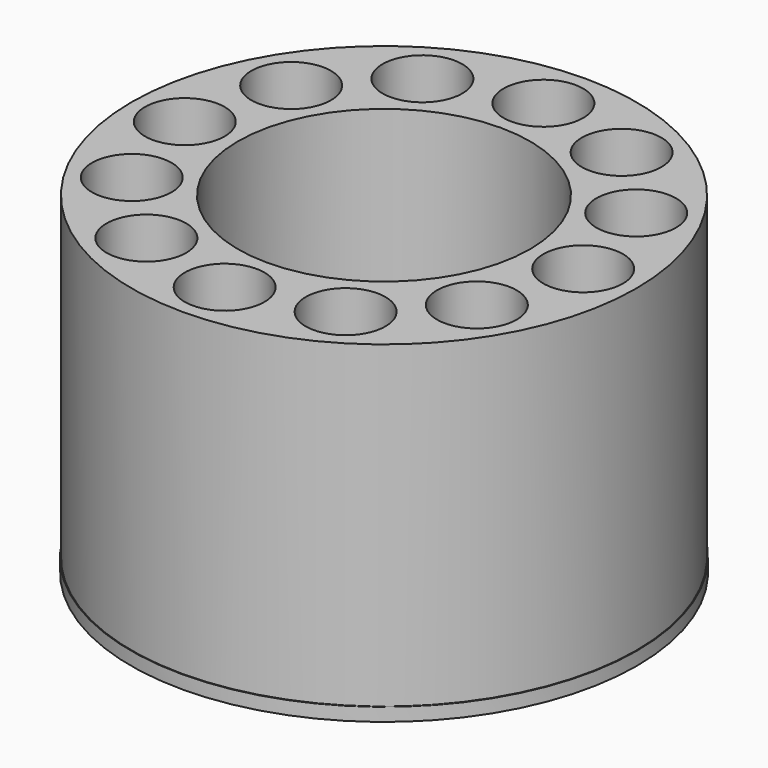
from build123d import *

# Parameters (mm, degrees)
F0_R     = 30.1625
F0_R_2   = 4.7625
F0_R_3   = 17.4625
F1_DEPTH = 38.1
F2_R     = 30.2476554836
F3_DEPTH = 1.5875


with BuildPart() as f1:
    # F0 (on Top) → F1 (new body)
    with BuildSketch(Plane.XY):
        Circle(F0_R)
        with Locations((-11.90625, -20.6222299276)):
            Circle(F0_R_2, mode=Mode.SUBTRACT)
        with Locations((-20.6222299276, -11.90625)):
            Circle(F0_R_2, mode=Mode.SUBTRACT)
        with Locations((0, -23.8125)):
            Circle(F0_R_2, mode=Mode.SUBTRACT)
        with Locations((11.90625, -20.6222299276)):
            Circle(F0_R_2, mode=Mode.SUBTRACT)
        with Locations((20.6222299276, -11.90625)):
            Circle(F0_R_2, mode=Mode.SUBTRACT)
        with Locations((-23.8125, 0)):
            Circle(F0_R_2, mode=Mode.SUBTRACT)
        with Locations((-20.6222299276, 11.90625)):
            Circle(F0_R_2, mode=Mode.SUBTRACT)
        with Locations((-11.90625, 20.6222299276)):
            Circle(F0_R_2, mode=Mode.SUBTRACT)
        Circle(F0_R_3, mode=Mode.SUBTRACT)
        with Locations((23.8125, 0)):
            Circle(F0_R_2, mode=Mode.SUBTRACT)
        with Locations((20.6222299276, 11.90625)):
            Circle(F0_R_2, mode=Mode.SUBTRACT)
        with Locations((11.90625, 20.6222299276)):
            Circle(F0_R_2, mode=Mode.SUBTRACT)
        with Locations((0, 23.8125)):
            Circle(F0_R_2, mode=Mode.SUBTRACT)
    extrude(amount=F1_DEPTH)

    # F2 (on face) → F3 (join)
    with BuildSketch(Plane(origin=(0, 0, 0), x_dir=(1, 0, 0), z_dir=(0, 0, -1))):
        Circle(F2_R)
    extrude(amount=F3_DEPTH)


solid = f1.part
